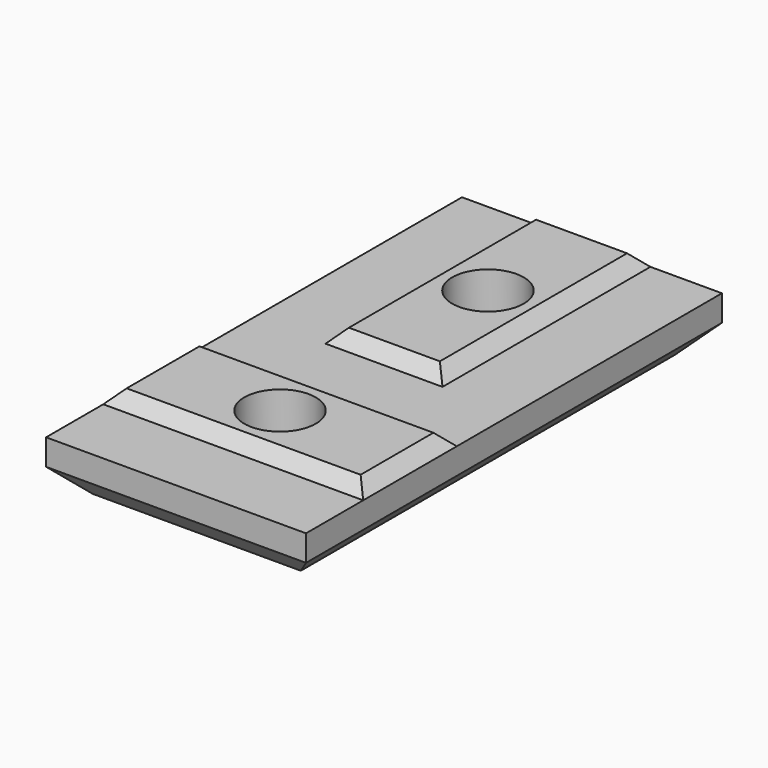
from build123d import *

# Parameters (mm, degrees)
F0_W     = 20
F0_H     = 40
F1_DEPTH = 4
F2_W     = 9
F2_H     = 20
F2_W_2   = 20
F2_H_2   = 9
F3_DEPTH = 1
F4_SIZE  = 0.99999
F5_R     = 2.75
F6_DEPTH = 5.001
F7_SIZE  = 2


# Not quite as in the source:
# - a fillet or chamfer is up to 0.001 mm smaller than in the source, because OpenCascade refuses the exact size


with BuildPart() as f1:
    # F0 (on Top) → F1 (new body)
    with BuildSketch(Plane.XY):
        with Locations((10, 20)):
            Rectangle(F0_W, F0_H)
    extrude(amount=F1_DEPTH)

    # F2 (on face) → F3 (join)
    with BuildSketch(Plane.XY.offset(4)):
        with Locations((10, 30)):
            Rectangle(F2_W, F2_H)
        with Locations((10, 10)):
            Rectangle(F2_W_2, F2_H_2)
    extrude(amount=F3_DEPTH)

    # F4 (size 1 in the source; OpenCascade refuses exactly that, so slightly less here)
    f4_edges = [f1.edges().sort_by_distance(p)[0] for p in [
        (10, 40, 5),
        (5.5, 30, 5),
        (10, 20, 5),
        (14.5, 30, 5),
        (10, 14.5, 5),
        (0, 10, 5),
        (10, 5.5, 5),
        (20, 10, 5),
    ]]
    chamfer(f4_edges, length=F4_SIZE)

    # F5 (on face) → F6 (cut, through all)
    with BuildSketch(Plane.XY.offset(5)):
        with Locations((10, 30)):
            Circle(F5_R)
        with Locations((10, 10)):
            Circle(F5_R)
    extrude(amount=-F6_DEPTH, mode=Mode.SUBTRACT)

    # F7
    f7_edges = [f1.edges().sort_by_distance(p)[0] for p in [
        (0, 20, 0),
        (10, 0, 0),
        (20, 20, 0),
        (10, 40, 0),
    ]]
    chamfer(f7_edges, length=F7_SIZE)


solid = f1.part
